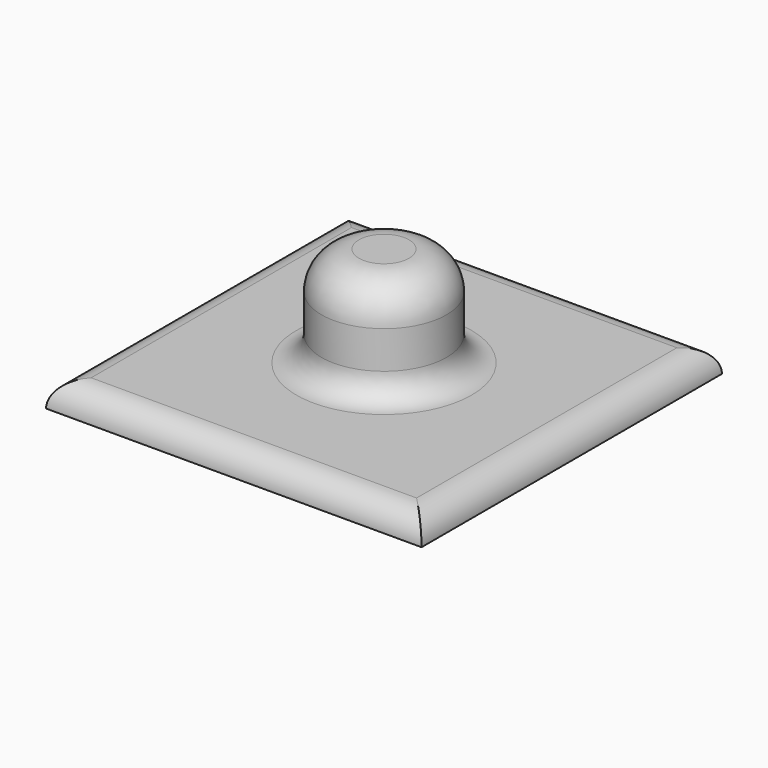
from build123d import *

# Parameters (mm, degrees)
F0_W     = 30
F0_H     = 30
F1_DEPTH = 2
F2_R     = 5
F3_DEPTH = 8
F4_R     = 3
F5_R     = 1.99999


# Not quite as in the source:
# - a fillet or chamfer is up to 0.001 mm smaller than in the source, because OpenCascade refuses the exact size


with BuildPart() as f1:
    # F0 (on Top) → F1 (new body)
    with BuildSketch(Plane.XY):
        Rectangle(F0_W, F0_H)
    extrude(amount=F1_DEPTH)

    # F2 (on face) → F3 (join)
    with BuildSketch(Plane.XY.offset(2)):
        Circle(F2_R)
    extrude(amount=F3_DEPTH)

    # F4
    f4_edges = [f1.edges().sort_by_distance(p)[0] for p in [
        (-5, 0, 10),
    ]]
    fillet(f4_edges, radius=F4_R)

    # F5 (radius 2 in the source; OpenCascade refuses exactly that, so slightly less here)
    f5_edges = [f1.edges().sort_by_distance(p)[0] for p in [
        (0, -15, 2),
        (-15, 0, 2),
        (15, 0, 2),
        (0, 15, 2),
        (-5, 0, 2),
    ]]
    fillet(f5_edges, radius=F5_R)


solid = f1.part
